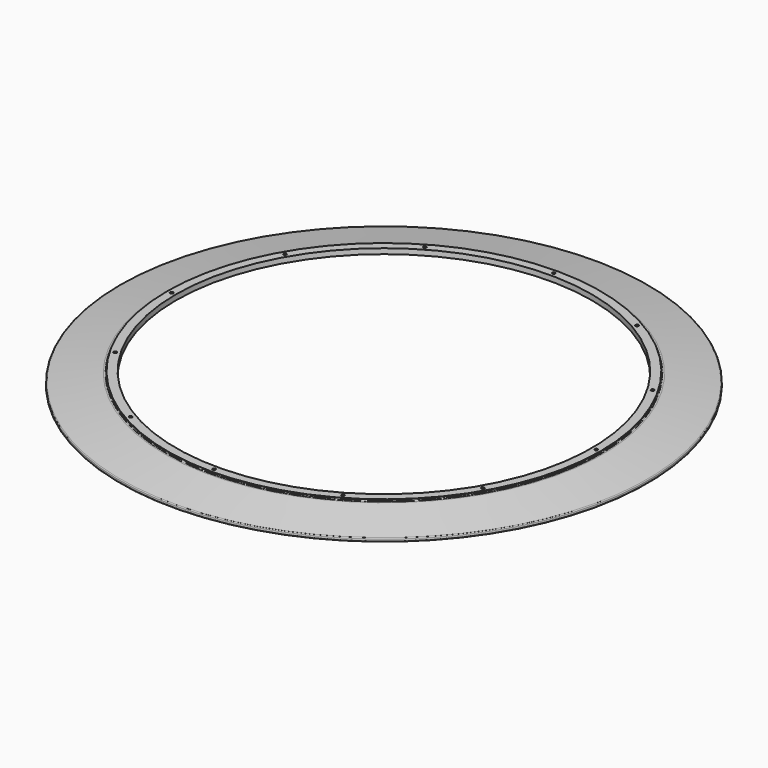
from build123d import *

# Parameters (mm, degrees)
F3_D            = 7
F3_DEPTH        = 50
F3_CBORE_D      = 11
F3_CBORE_DEPTH  = 3
F3_TIP          = 2.1030121666
F3_COPIES_COUNT = 12
F4_R            = 2


# Not quite as in the source:
# - a pattern or mirror of a feature is missing from the dataset's text; its kind, count and spacing are read off the source's solid


with BuildPart() as f1:
    # F0 (on Front) → F1 (revolve)
    with BuildSketch(Plane.XZ):
        with BuildLine():
            Line((-472.75, -12), (-472.75, 0))
            Line((-472.75, 0), (-492.5, 0))
            Line((-492.5, 0), (-492.5, -4))
            Line((-492.5, -4), (-498.1718563043, -4.1215379759))
            Line((-498.1718563043, -4.1215379759), (-598.3472963553, -21.7851708612))
            ThreePointArc((-598.3472963553, -21.7851708612), (-599.5320888862, -22.4692111479), (-600, -23.7547863673))
            Line((-600, -23.7547863673), (-600, -27.8164928148))
            ThreePointArc((-600, -27.8164928148), (-599.2855752194, -29.348581701), (-597.6527036447, -29.7861083208))
            Line((-597.6527036447, -29.7861083208), (-496.782670883, -12))
            Line((-496.782670883, -12), (-472.75, -12))
        make_face()
    revolve(axis=Axis((0, 0, -202.4746355881), (0, 0, -1)))

    # F3
    with Locations(Plane(origin=(0, 0, -12), x_dir=(1, 0, 0), z_dir=(0, 0, -1))):
        with Locations((0, -482.5)):
            f3 = CounterBoreHole(F3_D / 2, F3_CBORE_D / 2, F3_CBORE_DEPTH, depth=F3_DEPTH)
            with Locations((0, 0, -(F3_DEPTH + F3_TIP / 2))):  # 118° drill point
                Cone(0, F3_D / 2, F3_TIP, mode=Mode.SUBTRACT)

    # F3_copies: F3 ×12 about axis
    f3_copies_axis = Axis((0, 0, 0), (0, 0, 1))
    for i in range(1, F3_COPIES_COUNT):
        add(f3.rotate(f3_copies_axis, i * 360 / F3_COPIES_COUNT), mode=Mode.SUBTRACT)

    # F4
    f4_edges = [f1.edges().sort_by_distance(p)[0] for p in [
        (492.5, 0, -4),
    ]]
    fillet(f4_edges, radius=F4_R)


solid = f1.part
